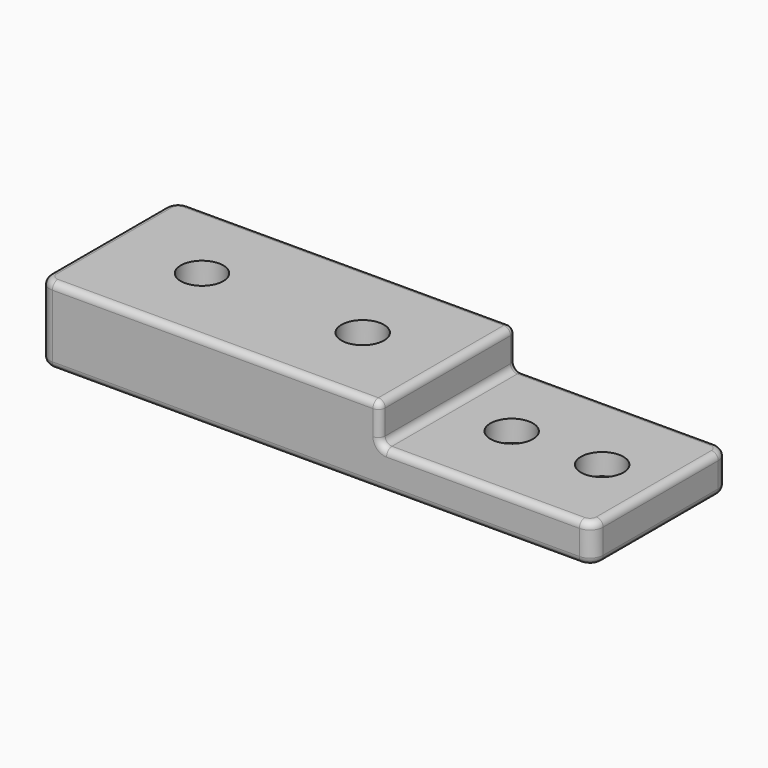
from build123d import *

# Parameters (mm, degrees)
F0_W          = 40.64
F0_H          = 20.32
F0_R          = 2.54
F1_DEPTH      = 9.144
F2_W          = 25.4
F2_H          = 20.32
F2_R          = 2.54
F3_DEPTH      = 4.572
F4_R          = 5.334
F4_R_2        = 2.54
F5_DEPTH      = 4.1148
F6_R          = 4.445
F6_R_2        = 2.54
F7_DEPTH      = 2.032
F8_R          = 1.5748
F9_F1_R       = 0.8128
F9_F2_R       = 0.8128
F10_T1_DEPTH  = 38.2524
F10_T3_DEPTH  = 62.8904
F10_T5_DEPTH  = 17.1704
F10_S9_W      = 0.8128
F10_S9_H      = 0.8128
F10_T10_DEPTH = 0.8128
F10_S15_W     = 0.8128
F10_S15_H     = 0.8128
F10_T16_DEPTH = 0.8128
F10_T20_ANGLE = 90
F10_T22_ANGLE = 90
F10_T24_ANGLE = 90
F10_T26_ANGLE = 90
F10_T28_ANGLE = 90
F10_T30_ANGLE = 90


# Not quite as in the source:
# - a fillet or chamfer that OpenCascade refuses, or shapes differently, is made with other operations: its cross-section is extruded or revolved along the edge and cut away or added


with BuildPart() as f1:
    # F0 (on Top) → F1 (new body)
    with BuildSketch(Plane.XY):
        with Locations((-20.32, 0)):
            Rectangle(F0_W, F0_H)
        with Locations((-29.337, 0)):
            Circle(F0_R, mode=Mode.SUBTRACT)
        with Locations((-10.16, 0)):
            Circle(F0_R, mode=Mode.SUBTRACT)
    extrude(amount=F1_DEPTH)

    # F2 (on Top) → F3 (join)
    with BuildSketch(Plane.XY):
        with Locations((12.7, 0)):
            Rectangle(F2_W, F2_H)
        with Locations((7.62, 0)):
            Circle(F2_R, mode=Mode.SUBTRACT)
        with Locations((18.415, 0)):
            Circle(F2_R, mode=Mode.SUBTRACT)
    extrude(amount=F3_DEPTH)

    # F4 (on face) → F5 (cut)
    with BuildSketch(Plane(origin=(0, 0, 0), x_dir=(1, 0, 0), z_dir=(0, 0, -1))):
        with Locations((-29.337, 0)):
            Circle(F4_R)
        with Locations((-29.337, 0)):
            Circle(F4_R_2, mode=Mode.SUBTRACT)
        with Locations((-10.16, 0)):
            Circle(F4_R)
        with Locations((-10.16, 0)):
            Circle(F4_R_2, mode=Mode.SUBTRACT)
    extrude(amount=-F5_DEPTH, mode=Mode.SUBTRACT)

    # F6 (on face) → F7 (cut)
    with BuildSketch(Plane(origin=(0, 0, 0), x_dir=(1, 0, 0), z_dir=(0, 0, -1))):
        with Locations((7.62, 0)):
            Circle(F6_R)
        with Locations((7.62, 0)):
            Circle(F6_R_2, mode=Mode.SUBTRACT)
        with Locations((18.415, 0)):
            Circle(F6_R)
        with Locations((18.415, 0)):
            Circle(F6_R_2, mode=Mode.SUBTRACT)
    extrude(amount=-F7_DEPTH, mode=Mode.SUBTRACT)

    # F8
    f8_edges = [f1.edges().sort_by_distance(p)[0] for p in [
        (-40.64, 10.16, 4.572),
        (-40.64, -10.16, 4.572),
        (25.4, 10.16, 2.286),
        (25.4, -10.16, 2.286),
    ]]
    fillet(f8_edges, radius=F8_R)

    # F9: fillet of radius 0.8128 on 3 edges, made by hand

    # F9_f1
    f9_f1_edges = [f1.edges().sort_by_distance(p)[0] for p in [
        (0, 0, 4.572),
    ]]
    fillet(f9_f1_edges, radius=F9_F1_R)

    # F9_f2
    f9_f2_edges = [f1.edges().sort_by_distance(p)[0] for p in [
        (0, 10.16, 7.2644),
        (0, 0, 9.144),
        (0.2380636083, 10.16, 4.8100636083),
    ]]
    fillet(f9_f2_edges, radius=F9_F2_R)

    # F10: fillet of radius 0.8128 on 13 edges, made by hand

    # F10_s2 → F10_t1 (cut)
    with BuildSketch(Plane.YZ.offset(-39.0652)):
        with BuildLine():
            ThreePointArc((-9.3472, 9.144), (-9.9219363917, 8.9059363917), (-10.16, 8.3312))
            Line((-10.16, 8.3312), (-10.16, 9.144))
            Line((-10.16, 9.144), (-9.3472, 9.144))
        make_face()
        with BuildLine():
            ThreePointArc((10.16, 8.3312), (9.9219363917, 8.9059363917), (9.3472, 9.144))
            Line((9.3472, 9.144), (10.16, 9.144))
            Line((10.16, 9.144), (10.16, 8.3312))
        make_face()
    extrude(amount=F10_T1_DEPTH, mode=Mode.SUBTRACT)

    # F10_s4 → F10_t3 (cut)
    with BuildSketch(Plane.YZ.offset(-39.0652)):
        with BuildLine():
            ThreePointArc((10.16, 0.8128), (9.9219363917, 0.2380636083), (9.3472, 0))
            Line((9.3472, 0), (10.16, 0))
            Line((10.16, 0), (10.16, 0.8128))
        make_face()
        with BuildLine():
            ThreePointArc((-9.3472, 0), (-9.9219363917, 0.2380636083), (-10.16, 0.8128))
            Line((-10.16, 0.8128), (-10.16, 0))
            Line((-10.16, 0), (-9.3472, 0))
        make_face()
    extrude(amount=F10_T3_DEPTH, mode=Mode.SUBTRACT)

    # F10_s6 → F10_t5 (cut)
    with BuildSketch(Plane.XZ.offset(-8.5852)):
        with BuildLine():
            ThreePointArc((-39.8272, 9.144), (-40.4019363917, 8.9059363917), (-40.64, 8.3312))
            Line((-40.64, 8.3312), (-40.64, 9.144))
            Line((-40.64, 9.144), (-39.8272, 9.144))
        make_face()
        with BuildLine():
            ThreePointArc((-39.8272, 0), (-40.4019363917, 0.2380636083), (-40.64, 0.8128))
            Line((-40.64, 0.8128), (-40.64, 0))
            Line((-40.64, 0), (-39.8272, 0))
        make_face()
        with BuildLine():
            ThreePointArc((24.5872, 0), (25.1619363917, 0.2380636083), (25.4, 0.8128))
            Line((25.4, 0.8128), (25.4, 0))
            Line((25.4, 0), (24.5872, 0))
        make_face()
    extrude(amount=F10_T5_DEPTH, mode=Mode.SUBTRACT)


with BuildPart() as f10_tool8:
    # F10_s9 → F10_t10 (new body)
    with BuildSketch(Plane.XZ.offset(-9.3472)):
        with Locations((-0.4064, 8.7376)):
            Rectangle(F10_S9_W, F10_S9_H)
    extrude(amount=-F10_T10_DEPTH)

    # F10_s11 → F10_t12 (revolve, cut)
    with BuildSketch(Plane(origin=(-0.8128, 9.3472, 8.3312), x_dir=(-0.7071067812, 0, -0.7071067812), z_dir=(0.7071067812, 0, -0.7071067812))):
        with BuildLine():
            ThreePointArc((0, -0.8128), (0.8128, 0), (0, 0.8128))
            Line((0, 0.8128), (0, -0.8128))
        make_face()
    revolve(axis=Axis((-0.8128, 9.3472, 8.3312), (0, 1, 0)), mode=Mode.SUBTRACT)


with BuildPart() as f1_1:
    add(f1.part)

    # F10_t7: cut F10_tool8
    add(f10_tool8.part, mode=Mode.SUBTRACT)


with BuildPart() as f10_tool14:
    # F10_s15 → F10_t16 (new body)
    with BuildSketch(Plane.XY.offset(8.3312)):
        with Locations((-0.4064, -9.7536)):
            Rectangle(F10_S15_W, F10_S15_H)
    extrude(amount=F10_T16_DEPTH)

    # F10_s17 → F10_t18 (revolve, cut)
    with BuildSketch(Plane(origin=(-0.8128, -9.3472, 8.3312), x_dir=(-0.7071067812, 0.7071067812, 0), z_dir=(0.7071067812, 0.7071067812, 0))):
        with BuildLine():
            ThreePointArc((0, -0.8128), (0.8128, 0), (0, 0.8128))
            Line((0, 0.8128), (0, -0.8128))
        make_face()
    revolve(axis=Axis((-0.8128, -9.3472, 8.3312), (0, 0, 1)), mode=Mode.SUBTRACT)


with BuildPart() as f1_2:
    add(f1_1.part)

    # F10_t13: cut F10_tool14
    add(f10_tool14.part, mode=Mode.SUBTRACT)

    # F10_s19 → F10_t20 (revolve, cut)
    with BuildSketch(Plane.YZ.offset(-39.0652)):
        with BuildLine():
            ThreePointArc((9.3472, 9.144), (9.9219363917, 8.9059363917), (10.16, 8.3312))
            Line((10.16, 8.3312), (10.16, 9.144))
            Line((10.16, 9.144), (9.3472, 9.144))
        make_face()
    revolve(axis=Axis((-39.0652, 8.5852, 9.144), (0, 0, 1)), revolution_arc=F10_T20_ANGLE, mode=Mode.SUBTRACT)

    # F10_s21 → F10_t22 (revolve, cut)
    with BuildSketch(Plane.XZ.offset(8.5852)):
        with BuildLine():
            ThreePointArc((-39.8272, 9.144), (-40.4019363917, 8.9059363917), (-40.64, 8.3312))
            Line((-40.64, 8.3312), (-40.64, 9.144))
            Line((-40.64, 9.144), (-39.8272, 9.144))
        make_face()
    revolve(axis=Axis((-39.0652, -8.5852, 9.144), (0, 0, 1)), revolution_arc=F10_T22_ANGLE, mode=Mode.SUBTRACT)

    # F10_s23 → F10_t24 (revolve, cut)
    with BuildSketch(Plane.YZ.offset(-39.0652)):
        with BuildLine():
            ThreePointArc((10.16, 0.8128), (9.9219363917, 0.2380636083), (9.3472, 0))
            Line((9.3472, 0), (10.16, 0))
            Line((10.16, 0), (10.16, 0.8128))
        make_face()
    revolve(axis=Axis((-39.0652, 8.5852, 0), (0, 0, 1)), revolution_arc=F10_T24_ANGLE, mode=Mode.SUBTRACT)

    # F10_s25 → F10_t26 (revolve, cut)
    with BuildSketch(Plane.XZ.offset(8.5852)):
        with BuildLine():
            ThreePointArc((-39.8272, 0), (-40.4019363917, 0.2380636083), (-40.64, 0.8128))
            Line((-40.64, 0.8128), (-40.64, 0))
            Line((-40.64, 0), (-39.8272, 0))
        make_face()
    revolve(axis=Axis((-39.0652, -8.5852, 0), (0, 0, 1)), revolution_arc=F10_T26_ANGLE, mode=Mode.SUBTRACT)

    # F10_s27 → F10_t28 (revolve, cut)
    with BuildSketch(Plane.YZ.offset(23.8252)):
        with BuildLine():
            ThreePointArc((9.3472, 0), (9.9219363917, 0.2380636083), (10.16, 0.8128))
            Line((10.16, 0.8128), (10.16, 0))
            Line((10.16, 0), (9.3472, 0))
        make_face()
    revolve(axis=Axis((23.8252, 8.5852, 0), (0, 0, -1)), revolution_arc=F10_T28_ANGLE, mode=Mode.SUBTRACT)

    # F10_s29 → F10_t30 (revolve, cut)
    with BuildSketch(Plane.XZ.offset(8.5852)):
        with BuildLine():
            ThreePointArc((24.5872, 0), (25.1619363917, 0.2380636083), (25.4, 0.8128))
            Line((25.4, 0.8128), (25.4, 0))
            Line((25.4, 0), (24.5872, 0))
        make_face()
    revolve(axis=Axis((23.8252, -8.5852, 0), (0, 0, -1)), revolution_arc=F10_T30_ANGLE, mode=Mode.SUBTRACT)


solid = f1_2.part
